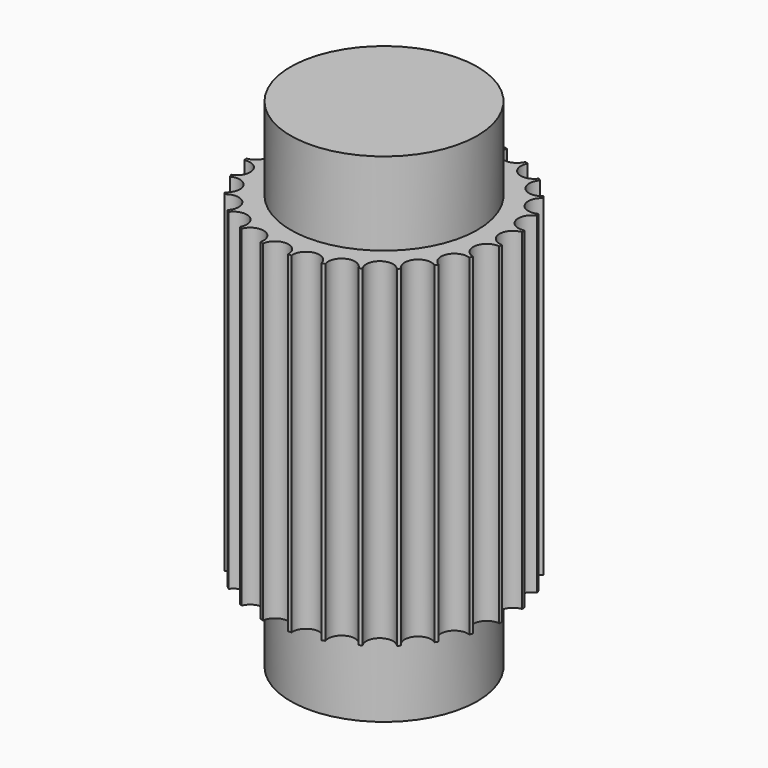
from build123d import *

# Parameters (mm, degrees)
F2_DEPTH      = 101.6
F3_R          = 28.575
F4_DEPTH      = 25.4
F4_DEPTH_BACK = 127


# Not quite as in the source:
# - a variable given as a bare number and used for a length is read in inches; the dataset says mm whatever the document's units were


with BuildPart() as f2:
    # F1 (on Top) → F2 (new body)
    with BuildSketch(Plane.XY):
        with BuildLine():
            ThreePointArc((38.0275754542, -2.3480854065), (33.9582141815, 1.5680199369), (37.6493768268, 5.8424673345))
            ThreePointArc((37.6493768268, 5.8424673345), (37.5682491535, 6.3432369925), (37.4804611085, 6.8428820754))
            ThreePointArc((37.4804611085, 6.8428820754), (32.5904927394, 9.6684424763), (35.1484807634, 14.703547192))
            ThreePointArc((35.1484807634, 14.703547192), (34.949592771, 15.1702328637), (34.7445086614, 15.6342290466))
            ThreePointArc((34.7445086614, 15.6342290466), (29.3195046315, 17.2042333476), (30.5949329549, 22.705948064))
            ThreePointArc((30.5949329549, 22.705948064), (30.2898995917, 23.1112955656), (29.9794962155, 23.5125457292))
            ThreePointArc((29.9794962155, 23.5125457292), (24.3362737456, 23.7353065516), (24.254658063, 29.3823341865))
            ThreePointArc((24.254658063, 29.3823341865), (23.861293108, 29.7026714491), (23.4636978498, 30.0177428068))
            ThreePointArc((23.4636978498, 30.0177428068), (17.9318179962, 28.8802510423), (16.4979246183, 34.3428083198))
            ThreePointArc((16.4979246183, 34.3428083198), (16.0392003661, 34.5594278254), (15.5776325681, 34.7699203849))
            ThreePointArc((15.5776325681, 34.7699203849), (10.4801540403, 32.3386049206), (7.7777215434, 37.2976815311))
            ThreePointArc((7.7777215434, 37.2976815311), (7.2804272356, 37.3979328208), (6.7818422008, 37.4915539337))
            ThreePointArc((6.7818422008, 37.4915539337), (2.4164549121, 33.9084022415), (-1.3966961475, 38.0743908667))
            ThreePointArc((-1.3966961475, 38.0743908667), (-1.611243941, 38.0659151074), (-1.8257405619, 38.0562303887))
            ThreePointArc((-1.8257405619, 38.0562303887), (-1.8097889216, 37.8477980327), (-1.8044671093, 37.638823919))
            ThreePointArc((-1.8044671093, 37.638823919), (-5.4804796414, 33.5557575077), (-9.9257732847, 36.7843584245))
            ThreePointArc((-9.9257732847, 36.7843584245), (-10.4146635829, 36.648939718), (-10.901707494, 36.5070236217))
            ThreePointArc((-10.901707494, 36.5070236217), (-10.7216553993, 35.8248982817), (-10.661041443, 35.1220187156))
            ThreePointArc((-10.661041443, 35.1220187156), (-13.8468450451, 31.1207754191), (-18.4601131844, 33.3291797262))
            ThreePointArc((-18.4601131844, 33.3291797262), (-18.9022425388, 33.0804357137), (-19.3410207665, 32.8258269616))
            ThreePointArc((-19.3410207665, 32.8258269616), (-18.8304314471, 31.7405924789), (-18.6552519207, 30.5541071359))
            ThreePointArc((-18.6552519207, 30.5541071359), (-21.3643249191, 26.6933193437), (-25.9163927322, 27.9275954524))
            ThreePointArc((-25.9163927322, 27.9275954524), (-26.2859410341, 27.580052646), (-26.6508291737, 27.2276202478))
            ThreePointArc((-26.6508291737, 27.2276202478), (-25.6675808238, 25.8545575842), (-25.3202410927, 24.2018526781))
            ThreePointArc((-25.3202410927, 24.2018526781), (-27.5730476059, 20.5380946086), (-31.8591693457, 20.8950551232))
            ThreePointArc((-31.8591693457, 20.8950551232), (-32.1345551797, 20.4690098296), (-32.4042439666, 20.0393356415))
            ThreePointArc((-32.4042439666, 20.0393356415), (-30.8413491085, 18.5309299599), (-30.266777295, 16.4362234724))
            ThreePointArc((-30.266777295, 16.4362234724), (-32.090467362, 13.0231821609), (-35.9413881732, 12.6422551859))
            ThreePointArc((-35.9413881732, 12.6422551859), (-36.1065291595, 12.1625882135), (-36.2652689185, 11.6807649693))
            ThreePointArc((-36.2652689185, 11.6807649693), (-34.0595315808, 10.2167411474), (-33.2059855622, 7.7107279494))
            ThreePointArc((-33.2059855622, 7.7107279494), (-34.633997298, 4.5984165422), (-37.9246499035, 3.6511545708))
            ThreePointArc((-37.9246499035, 3.6511545708), (-37.9699019004, 3.1458782044), (-38.0084223177, 2.6400441138))
            ThreePointArc((-38.0084223177, 2.6400441138), (-35.1463921507, 1.415528136), (-33.9662177648, -1.4650698011))
            ThreePointArc((-33.9662177648, -1.4650698011), (-35.0377873736, -4.231044916), (-37.6931331536, -5.5531714423))
            ThreePointArc((-37.6931331536, -5.5531714423), (-37.6158534696, -6.0545493438), (-37.5319049742, -6.554853851))
            ThreePointArc((-37.5319049742, -6.554853851), (-34.0527474172, -7.3423365778), (-32.5030767644, -10.5553082894))
            ThreePointArc((-32.5030767644, -10.5553082894), (-33.2626635907, -12.9344157776), (-35.2603583731, -14.4331953289))
            ThreePointArc((-35.2603583731, -14.4331953289), (-35.0650600987, -14.9013945747), (-34.8635452362, -15.3669519932))
            ThreePointArc((-34.8635452362, -15.3669519932), (-30.8586295725, -15.530858571), (-28.9020091826, -19.029122639))
            ThreePointArc((-28.9020091826, -19.029122639), (-29.3986442237, -20.9865001474), (-30.7683982573, -22.4703286287))
            ThreePointArc((-30.7683982573, -22.4703286287), (-30.4664867033, -22.878006643), (-30.1591738296, -23.2816286783))
            ThreePointArc((-30.1591738296, -23.2816286783), (-25.7683757069, -22.6593523381), (-23.373315365, -26.3916468007))
            ThreePointArc((-23.373315365, -26.3916468007), (-23.6598827933, -27.8986118146), (-24.4795807808, -29.1952072231))
            ThreePointArc((-24.4795807808, -29.1952072231), (-24.0886874142, -29.5185558363), (-23.6935234304, -29.8366711859))
            ThreePointArc((-23.6935234304, -29.8366711859), (-19.0984337687, -28.3012799336), (-16.2398679583, -32.2129134548))
            ThreePointArc((-16.2398679583, -32.2129134548), (-16.3723301811, -33.2473835979), (-16.7611693897, -34.2151019389))
            ThreePointArc((-16.7611693897, -34.2151019389), (-16.3041221659, -34.4352377718), (-15.844184429, -34.649268676))
            ThreePointArc((-15.844184429, -34.649268676), (-11.2586011252, -32.1193105722), (-7.9182563272, -36.1529638633))
            ThreePointArc((-7.9182563272, -36.1529638633), (-7.9548339389, -36.6997804834), (-8.0639150202, -37.2368537144))
            ThreePointArc((-8.0639150202, -37.2368537144), (-7.567405243, -37.3409209566), (-7.0695538613, -37.4383681295))
            ThreePointArc((-7.0695538613, -37.4383681295), (-2.7277955027, -33.8851355215), (1.1055420333, -37.9817012719))
            ThreePointArc((1.1055420333, -37.9817012719), (1.105223389, -38.0328515683), (1.1042675055, -38.083993925))
            ThreePointArc((1.1042675055, -38.083993925), (1.611243941, -38.0659151074), (2.1179347234, -38.0410876883))
            ThreePointArc((2.1179347234, -38.0410876883), (5.5309497632, -33.5414309717), (10.2079614225, -36.707050053))
            ThreePointArc((10.2079614225, -36.707050053), (10.6957973741, -36.5678809686), (11.1817370971, -36.4222288649))
            ThreePointArc((11.1817370971, -36.4222288649), (13.4156740687, -31.2352154819), (18.7155160648, -33.1864348556))
            ThreePointArc((18.7155160648, -33.1864348556), (19.1557221841, -32.9343029015), (19.592532238, -32.6763321152))
            ThreePointArc((19.592532238, -32.6763321152), (20.5169304634, -27.1048807648), (26.1300949689, -27.7277503039))
            ThreePointArc((26.1300949689, -27.7277503039), (26.4969634631, -27.377379846), (26.8591343834, -27.0221557277))
            ThreePointArc((26.8591343834, -27.0221557277), (26.4200095201, -21.3916360729), (32.018690847, -20.6497805423))
            ThreePointArc((32.018690847, -20.6497805423), (32.2907967999, -20.2216330208), (32.5571780061, -19.7899004616))
            ThreePointArc((32.5571780061, -19.7899004616), (30.780174702, -14.4291317214), (36.0374129719, -12.3658750718))
            ThreePointArc((36.0374129719, -12.3658750718), (36.1988655471, -11.8849540641), (36.3539005248, -11.4019260055))
            ThreePointArc((36.3539005248, -11.4019260055), (33.3427947854, -6.6239740954), (37.9515702047, -3.3598093687))
            ThreePointArc((37.9515702047, -3.3598093687), (37.9929406615, -2.8542003943), (38.0275754542, -2.3480854065))
        make_face()
    extrude(amount=F2_DEPTH)

    # F3 (on face) → F4 (join, two sides)
    with BuildSketch(Plane(origin=(0, 0, 0), x_dir=(1, 0, 0), z_dir=(0, 0, -1))) as f4_sk:
        Circle(F3_R)
    extrude(amount=F4_DEPTH)
    extrude(f4_sk.sketch, amount=-F4_DEPTH_BACK)


solid = f2.part
